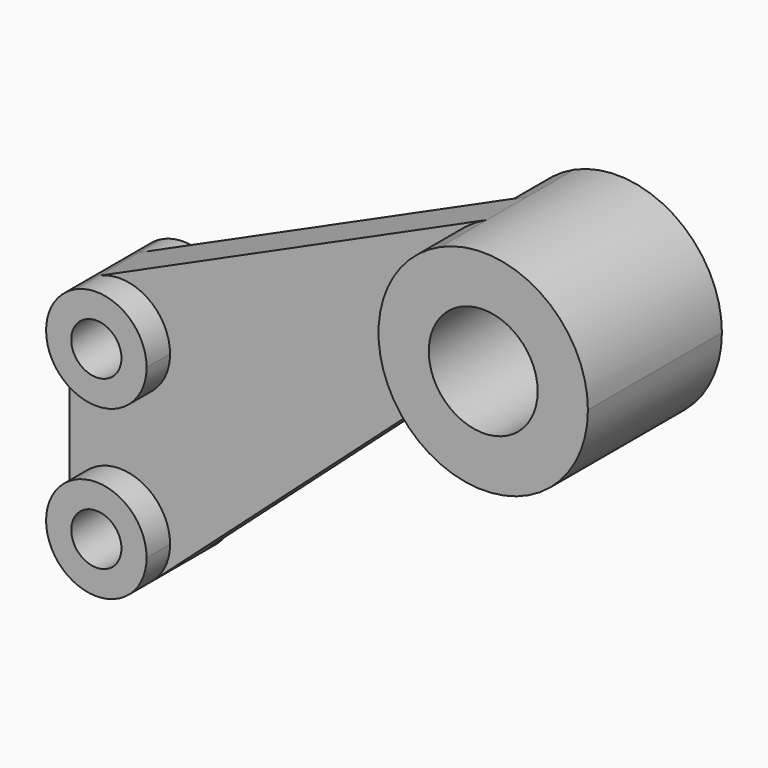
from build123d import *

# Parameters (mm, degrees)
F1_DEPTH = 5.9944
F0_R     = 5.9944
F2_DEPTH = 13.0048
F0_R_2   = 13.0048
F3_DEPTH = 20.0025


with BuildPart() as f1:
    # F0 (on Front) → F1 (new body, symmetric)
    with BuildSketch(Plane.XZ):
        with BuildLine():
            ThreePointArc((-12.949346, -21.392276), (-24.961282, 1.499814), (-10.294693, 22.788908))
            Line((-10.294693, 22.788908), (-102.934025, -19.060113))
            ThreePointArc((-102.934025, -19.060113), (-91.484026, -19.914411), (-85.9917, -29.9974))
            ThreePointArc((-85.9917, -29.9974), (-97.9932, -41.9989), (-109.9947, -29.9974))
            Line((-109.9947, -29.9974), (-109.9947, -70.0024))
            ThreePointArc((-109.9947, -70.0024), (-97.9932, -58.0009), (-85.9917, -70.0024))
            ThreePointArc((-85.9917, -70.0024), (-87.036779, -74.90065), (-89.990008, -78.945829))
            Line((-89.990008, -78.945829), (-27.152389, -22.714435))
            ThreePointArc((-27.152389, -22.714435), (-20.268898, -19.711211), (-12.949346, -21.392276))
        make_face()
    extrude(amount=F1_DEPTH, both=True)

    # F0 (on Front) → F2 (join, symmetric)
    with BuildSketch(Plane.XZ):
        with BuildLine():
            ThreePointArc((-109.9947, -70.0024), (-102.89145, -80.958821), (-89.990008, -78.945829))
            ThreePointArc((-89.990008, -78.945829), (-87.036779, -74.90065), (-85.9917, -70.0024))
            ThreePointArc((-85.9917, -70.0024), (-97.9932, -58.0009), (-109.9947, -70.0024))
        make_face()
        with Locations((-97.9932, -70.0024)):
            Circle(F0_R, mode=Mode.SUBTRACT)
        with BuildLine():
            ThreePointArc((-85.9917, -29.9974), (-91.484026, -19.914411), (-102.934025, -19.060113))
            ThreePointArc((-102.934025, -19.060113), (-108.076189, -23.488226), (-109.9947, -29.9974))
            ThreePointArc((-109.9947, -29.9974), (-97.9932, -41.9989), (-85.9917, -29.9974))
        make_face()
        with Locations((-97.9932, -29.9974)):
            Circle(F0_R, mode=Mode.SUBTRACT)
    extrude(amount=F2_DEPTH, both=True)

    # F0 (on Front) → F3 (join, symmetric)
    with BuildSketch(Plane.XZ):
        with BuildLine():
            ThreePointArc((-12.949346, -21.392276), (12.278025, -21.784516), (25.0063, 0))
            ThreePointArc((25.0063, 0), (13.562501, 21.008894), (-10.294693, 22.788908))
            ThreePointArc((-10.294693, 22.788908), (-24.961282, 1.499814), (-12.949346, -21.392276))
        make_face()
        Circle(F0_R_2, mode=Mode.SUBTRACT)
    extrude(amount=F3_DEPTH, both=True)


solid = f1.part
